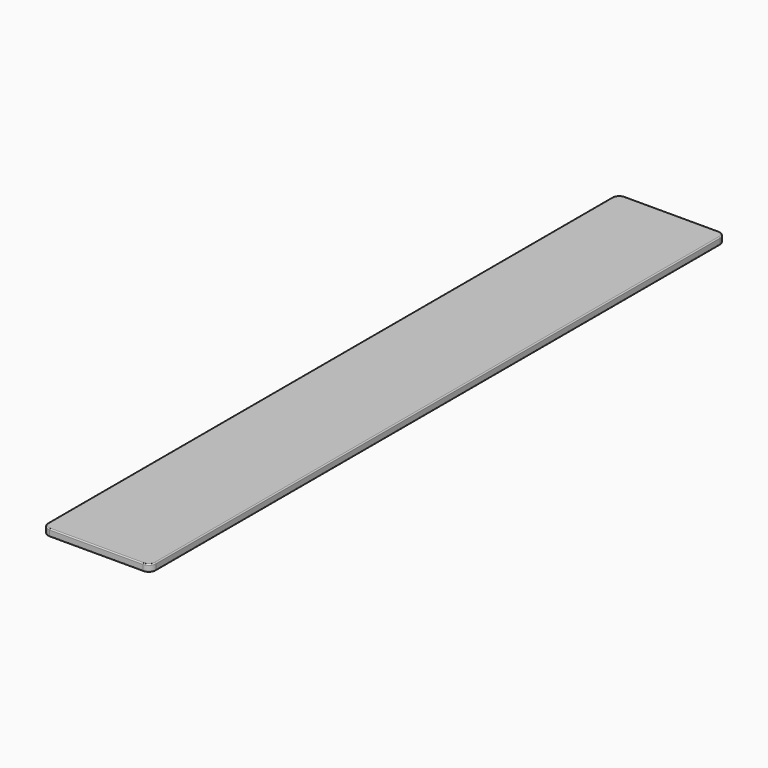
from build123d import *

# Parameters (mm, degrees)
F0_W         = 300
F0_H         = 20
F1_DEPTH     = 2000
F2_R         = 3
F3_T1_DEPTH  = 20
F3_T4_ANGLE  = 90
F3_T6_ANGLE  = 90
F3_T8_ANGLE  = 90
F3_T10_ANGLE = 90
F3_T12_ANGLE = 90
F3_T14_ANGLE = 90
F3_T16_ANGLE = 90
F3_T18_ANGLE = 90


# Not quite as in the source:
# - a fillet or chamfer that OpenCascade refuses, or shapes differently, is made with other operations: its cross-section is extruded or revolved along the edge and cut away or added


with BuildPart() as f1:
    # F0 (on Front) → F1 (new body)
    with BuildSketch(Plane.XZ):
        with Locations((66.0526476468, 10)):
            Rectangle(F0_W, F0_H)
    extrude(amount=F1_DEPTH)

    # F2
    f2_edges = [f1.edges().sort_by_distance(p)[0] for p in [
        (216.052648, -1000, 20),
        (-83.947352, -1000, 20),
        (66.052648, 0, 20),
        (66.052648, -2000, 20),
        (-83.947352, -1000, 0),
        (216.052648, -1000, 0),
        (66.052648, 0, 0),
        (66.052648, -2000, 0),
    ]]
    fillet(f2_edges, radius=F2_R)

    # F3: fillet of radius 20 on 4 edges, made by hand

    # F3_s2 → F3_t1 (cut)
    with BuildSketch(Plane.XY):
        with BuildLine():
            ThreePointArc((216.0526476468, -20), (210.1947832705, -5.8578643763), (196.0526476468, 0))
            Line((196.0526476468, 0), (216.0526476468, 0))
            Line((216.0526476468, 0), (216.0526476468, -20))
        make_face()
        with BuildLine():
            ThreePointArc((-63.9473523532, 0), (-78.0894879769, -5.8578643763), (-83.9473523532, -20))
            Line((-83.9473523532, -20), (-83.9473523532, 0))
            Line((-83.9473523532, 0), (-63.9473523532, 0))
        make_face()
        with BuildLine():
            ThreePointArc((216.0526476468, -1980), (210.1947832705, -1994.1421356237), (196.0526476468, -2000))
            Line((196.0526476468, -2000), (216.0526476468, -2000))
            Line((216.0526476468, -2000), (216.0526476468, -1980))
        make_face()
        with BuildLine():
            ThreePointArc((-63.9473523532, -2000), (-78.0894879769, -1994.1421356237), (-83.9473523532, -1980))
            Line((-83.9473523532, -1980), (-83.9473523532, -2000))
            Line((-83.9473523532, -2000), (-63.9473523532, -2000))
        make_face()
    extrude(amount=F3_T1_DEPTH, mode=Mode.SUBTRACT)

    # F3_s3 → F3_t4 (revolve, cut)
    with BuildSketch(Plane.XZ.offset(1980)):
        with BuildLine():
            ThreePointArc((-80.9473523532, 20), (-83.0686726968, 19.1213203436), (-83.9473523532, 17))
            Line((-83.9473523532, 17), (-83.9473523532, 20))
            Line((-83.9473523532, 20), (-80.9473523532, 20))
        make_face()
    revolve(axis=Axis((-63.9473523532, -1980, 20), (0, 0, 1)), revolution_arc=F3_T4_ANGLE, mode=Mode.SUBTRACT)

    # F3_s5 → F3_t6 (revolve, cut)
    with BuildSketch(Plane.YZ.offset(-63.9473523532)):
        with BuildLine():
            ThreePointArc((-1997, 0), (-1999.1213203436, 0.8786796564), (-2000, 3))
            Line((-2000, 3), (-2000, 0))
            Line((-2000, 0), (-1997, 0))
        make_face()
    revolve(axis=Axis((-63.9473523532, -1980, 0), (0, 0, -1)), revolution_arc=F3_T6_ANGLE, mode=Mode.SUBTRACT)

    # F3_s7 → F3_t8 (revolve, cut)
    with BuildSketch(Plane.XZ.offset(1980)):
        with BuildLine():
            ThreePointArc((213.0526476468, 0), (215.1739679904, 0.8786796564), (216.0526476468, 3))
            Line((216.0526476468, 3), (216.0526476468, 0))
            Line((216.0526476468, 0), (213.0526476468, 0))
        make_face()
    revolve(axis=Axis((196.0526476468, -1980, 0), (0, 0, -1)), revolution_arc=F3_T8_ANGLE, mode=Mode.SUBTRACT)

    # F3_s9 → F3_t10 (revolve, cut)
    with BuildSketch(Plane.YZ.offset(196.0526476468)):
        with BuildLine():
            ThreePointArc((-1997, 20), (-1999.1213203436, 19.1213203436), (-2000, 17))
            Line((-2000, 17), (-2000, 20))
            Line((-2000, 20), (-1997, 20))
        make_face()
    revolve(axis=Axis((196.0526476468, -1980, 20), (0, 0, 1)), revolution_arc=F3_T10_ANGLE, mode=Mode.SUBTRACT)

    # F3_s11 → F3_t12 (revolve, cut)
    with BuildSketch(Plane.YZ.offset(-63.9473523532)):
        with BuildLine():
            ThreePointArc((-3, 20), (-0.8786796564, 19.1213203436), (0, 17))
            Line((0, 17), (0, 20))
            Line((0, 20), (-3, 20))
        make_face()
    revolve(axis=Axis((-63.9473523532, -20, 20), (0, 0, 1)), revolution_arc=F3_T12_ANGLE, mode=Mode.SUBTRACT)

    # F3_s13 → F3_t14 (revolve, cut)
    with BuildSketch(Plane.XZ.offset(20)):
        with BuildLine():
            ThreePointArc((-80.9473523532, 0), (-83.0686726968, 0.8786796564), (-83.9473523532, 3))
            Line((-83.9473523532, 3), (-83.9473523532, 0))
            Line((-83.9473523532, 0), (-80.9473523532, 0))
        make_face()
    revolve(axis=Axis((-63.9473523532, -20, 0), (0, 0, -1)), revolution_arc=F3_T14_ANGLE, mode=Mode.SUBTRACT)

    # F3_s15 → F3_t16 (revolve, cut)
    with BuildSketch(Plane.YZ.offset(196.0526476468)):
        with BuildLine():
            ThreePointArc((-3, 0), (-0.8786796564, 0.8786796564), (0, 3))
            Line((0, 3), (0, 0))
            Line((0, 0), (-3, 0))
        make_face()
    revolve(axis=Axis((196.0526476468, -20, 0), (0, 0, -1)), revolution_arc=F3_T16_ANGLE, mode=Mode.SUBTRACT)

    # F3_s17 → F3_t18 (revolve, cut)
    with BuildSketch(Plane.XZ.offset(20)):
        with BuildLine():
            ThreePointArc((213.0526476468, 20), (215.1739679904, 19.1213203436), (216.0526476468, 17))
            Line((216.0526476468, 17), (216.0526476468, 20))
            Line((216.0526476468, 20), (213.0526476468, 20))
        make_face()
    revolve(axis=Axis((196.0526476468, -20, 20), (0, 0, 1)), revolution_arc=F3_T18_ANGLE, mode=Mode.SUBTRACT)


solid = f1.part
